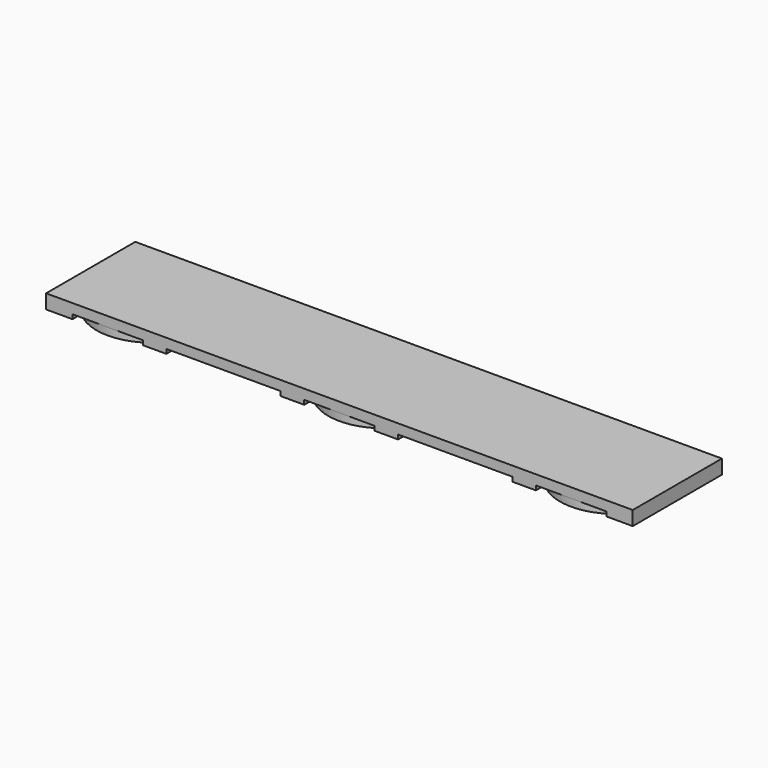
from build123d import *

# Parameters (mm, degrees)
F0_W     = 380
F0_H     = 33.5
F1_DEPTH = 1000
F3_DEPTH = 25
F4_R     = 4
F5_DEPTH = 15


# Not quite as in the source:
# - a feature names something its author has since deleted; it is built from what else it names


with BuildPart() as f1:
    # F0 (on Right) → F1 (new body, symmetric)
    with BuildSketch(Plane.YZ):
        with Locations((0, 16.75)):
            Rectangle(F0_W, F0_H)
    extrude(amount=F1_DEPTH, both=True)

    # F2 (on face) → F3 (join)
    with BuildSketch(Plane(origin=(0, 0, 0), x_dir=(1, 0, 0), z_dir=(0, 0, -1))):
        with BuildLine():
            ThreePointArc((-790, -190), (-655.6497115746, -134.3502884254), (-600, 0))
            ThreePointArc((-600, 0), (-655.6497118153, 134.3502886662), (-790.0000006809, 190))
            ThreePointArc((-790.0000006809, 190), (-980, -3.405e-07), (-790, -190))
        make_face()
        with BuildLine():
            ThreePointArc((190, 0), (134.350288533, 134.3502883179), (3.042e-07, 190))
            ThreePointArc((3.042e-07, 190), (-190, 1.521e-07), (0, -190))
            ThreePointArc((0, -190), (134.3502884254, -134.3502884254), (190, 0))
        make_face()
        with BuildLine():
            ThreePointArc((980, 0), (924.3502884254, 134.3502884254), (790, 190))
            ThreePointArc((790, 190), (600, 0), (790, -190))
            ThreePointArc((790, -190), (924.3502884254, -134.3502884254), (980, 0))
        make_face()
    extrude(amount=F3_DEPTH)

    # F4 (on face) → F5 (join)
    with BuildSketch(Plane(origin=(0, 0, 0), x_dir=(1, 0, 0), z_dir=(0, 0, -1))):
        Polygon((-990, 190), (-1000, 190), (-1000, 70), (-1000, -190), (-990, -190), (-990, -140), (-990, 140), align=None)
        Polygon((-910, 190), (-990, 190), (-990, 140), (-935.7230966807, 140), (-910, 166.1522239447), align=None)
        with Locations((-980, 180)):
            Circle(F4_R, mode=Mode.SUBTRACT)
        with Locations((-920, 180)):
            Circle(F4_R, mode=Mode.SUBTRACT)
        Polygon((-990, -140), (-990, -190), (-910, -190), (-910, -166.1522239447), (-935.7230966807, -140), align=None)
        with Locations((-980, -180)):
            Circle(F4_R, mode=Mode.SUBTRACT)
        with Locations((-920, -180)):
            Circle(F4_R, mode=Mode.SUBTRACT)
        Polygon((-590, 190), (-670, 190), (-670, 166.1522239447), (-644.2769033193, 140), (-590, 140), align=None)
        with Locations((-660, 180)):
            Circle(F4_R, mode=Mode.SUBTRACT)
        with Locations((-600, 180)):
            Circle(F4_R, mode=Mode.SUBTRACT)
        Polygon((-670, -166.1522239447), (-670, -190), (-590, -190), (-590, -140), (-644.2769033193, -140), align=None)
        with Locations((-660, -180)):
            Circle(F4_R, mode=Mode.SUBTRACT)
        with Locations((-600, -180)):
            Circle(F4_R, mode=Mode.SUBTRACT)
        Polygon((-120, 190), (-200, 190), (-200, 140), (-145.7230966807, 140), (-120, 166.1522239447), align=None)
        with Locations((-190, 180)):
            Circle(F4_R, mode=Mode.SUBTRACT)
        with Locations((-130, 180)):
            Circle(F4_R, mode=Mode.SUBTRACT)
        Polygon((-200, -140), (-200, -190), (-120, -190), (-120, -166.1522239447), (-145.7230966807, -140), align=None)
        with Locations((-190, -180)):
            Circle(F4_R, mode=Mode.SUBTRACT)
        with Locations((-130, -180)):
            Circle(F4_R, mode=Mode.SUBTRACT)
        Polygon((200, 190), (120, 190), (120, 166.1522239447), (145.7230966807, 140), (200, 140), align=None)
        with Locations((130, 180)):
            Circle(F4_R, mode=Mode.SUBTRACT)
        with Locations((190, 180)):
            Circle(F4_R, mode=Mode.SUBTRACT)
        Polygon((120, -166.1522239447), (120, -190), (200, -190), (200, -140), (145.7230966807, -140), align=None)
        with Locations((130, -180)):
            Circle(F4_R, mode=Mode.SUBTRACT)
        with Locations((190, -180)):
            Circle(F4_R, mode=Mode.SUBTRACT)
        Polygon((590, -140), (590, -190), (670, -190), (670, -166.1522239447), (644.2769033193, -140), align=None)
        with Locations((600, -180)):
            Circle(F4_R, mode=Mode.SUBTRACT)
        with Locations((660, -180)):
            Circle(F4_R, mode=Mode.SUBTRACT)
        Polygon((670, 190), (590, 190), (590, 140), (644.2769033193, 140), (670, 166.1522239447), align=None)
        with Locations((600, 180)):
            Circle(F4_R, mode=Mode.SUBTRACT)
        with Locations((660, 180)):
            Circle(F4_R, mode=Mode.SUBTRACT)
        Polygon((910, -166.1522239447), (910, -190), (990, -190), (990, -140), (935.7230966807, -140), align=None)
        with Locations((920, -180)):
            Circle(F4_R, mode=Mode.SUBTRACT)
        with Locations((980, -180)):
            Circle(F4_R, mode=Mode.SUBTRACT)
        Polygon((990, 190), (910, 190), (910, 166.1522239447), (935.7230966807, 140), (990, 140), align=None)
        with Locations((920, 180)):
            Circle(F4_R, mode=Mode.SUBTRACT)
        with Locations((980, 180)):
            Circle(F4_R, mode=Mode.SUBTRACT)
        Polygon((990, -140), (990, -190), (1000, -190), (1000, -70), (1000, 70), (1000, 190), (990, 190), (990, 140), align=None)
    extrude(amount=F5_DEPTH)


solid = f1.part
